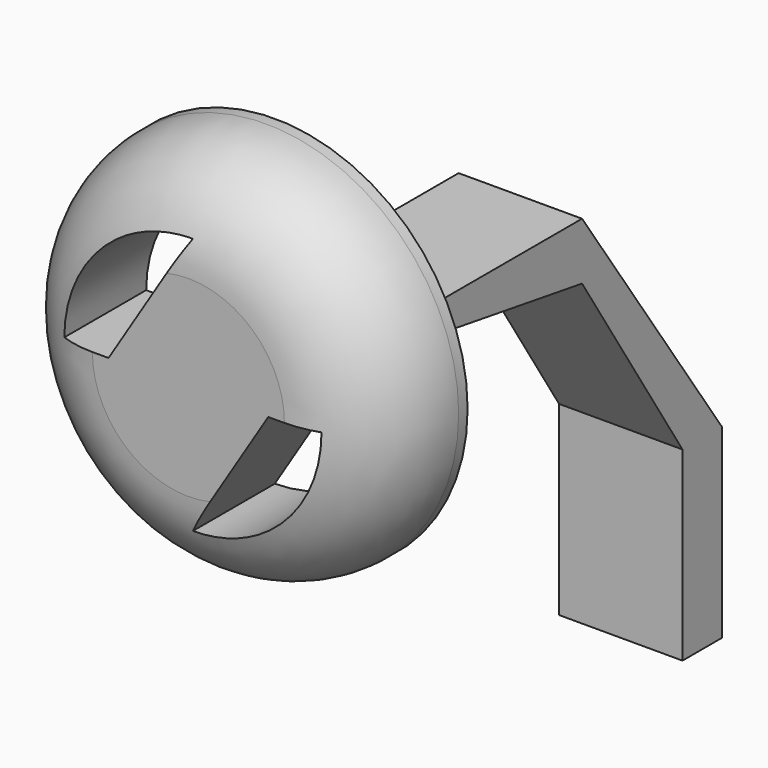
from build123d import *

# Parameters (mm, degrees)
F0_R     = 2.5
F2_DEPTH = 0.7
F3_DEPTH = 0.8


# Not quite as in the source:
# - a fillet or chamfer that OpenCascade refuses, or shapes differently, is made with other operations: its cross-section is extruded or revolved along the edge and cut away or added


with BuildPart() as f2:
    # F0 (on Front) → F2 (new body, symmetric)
    with BuildSketch(Plane.XZ):
        Circle(F0_R)
        with BuildLine():
            ThreePointArc((0, 1.6670872347), (1.1788086885, 1.1788086885), (1.6670872347, 0))
            ThreePointArc((1.6670872347, 0), (1.1788086885, -1.1788086885), (0, -1.6670872347))
            ThreePointArc((0, -1.6670872347), (-1.1788086885, -1.1788086885), (-1.6670872347, 0))
            ThreePointArc((-1.6670872347, 0), (-1.1788086885, 1.1788086885), (0, 1.6670872347))
        make_face(mode=Mode.SUBTRACT)
        Polygon((1.035158575, 0), (0, 1.6670872347), (-1.035158575, 0), (0, -1.6670872347), align=None)
        with BuildLine():
            Line((1.035158575, 0), (1.6670872347, 0))
            ThreePointArc((1.6670872347, 0), (1.1788086885, 1.1788086885), (0, 1.6670872347))
            Line((0, 1.6670872347), (1.035158575, 0))
        make_face()
        with BuildLine():
            ThreePointArc((-1.6670872347, 0), (-1.1788086885, -1.1788086885), (0, -1.6670872347))
            Line((0, -1.6670872347), (-1.035158575, 0))
            Line((-1.035158575, 0), (-1.6670872347, 0))
        make_face()
    extrude(amount=F2_DEPTH, both=True)

    # F1 (on Right) → F3 (join, symmetric)
    with BuildSketch(Plane.YZ):
        Polygon((4.6792123099, 0), (0, 0), (4.6792123099, -0.7401879564), (6.3069890554, -3.2957927736), (6.3069890554, -4.3182368269), (6.3069890554, -5.7057410895), (6.9458728476, -5.7057410895), (6.9458728476, -4.3182368269), (6.9458728476, -3.2957927736), align=None)
    extrude(amount=F3_DEPTH, both=True)

    # F4: fillet of radius 1.2553910524 on 1 edges, made by hand

    # F4_s1 → F4_t2 (revolve, cut)
    with BuildSketch(Plane.XY):
        with BuildLine():
            ThreePointArc((2.5, 0.5553910524), (2.1323044738, -0.3323044738), (1.2446089476, -0.7))
            Line((1.2446089476, -0.7), (2.5, -0.7))
            Line((2.5, -0.7), (2.5, 0.5553910524))
        make_face()
    revolve(axis=Axis((0, -0.7, 0), (0, -1, 0)), mode=Mode.SUBTRACT)


solid = f2.part
